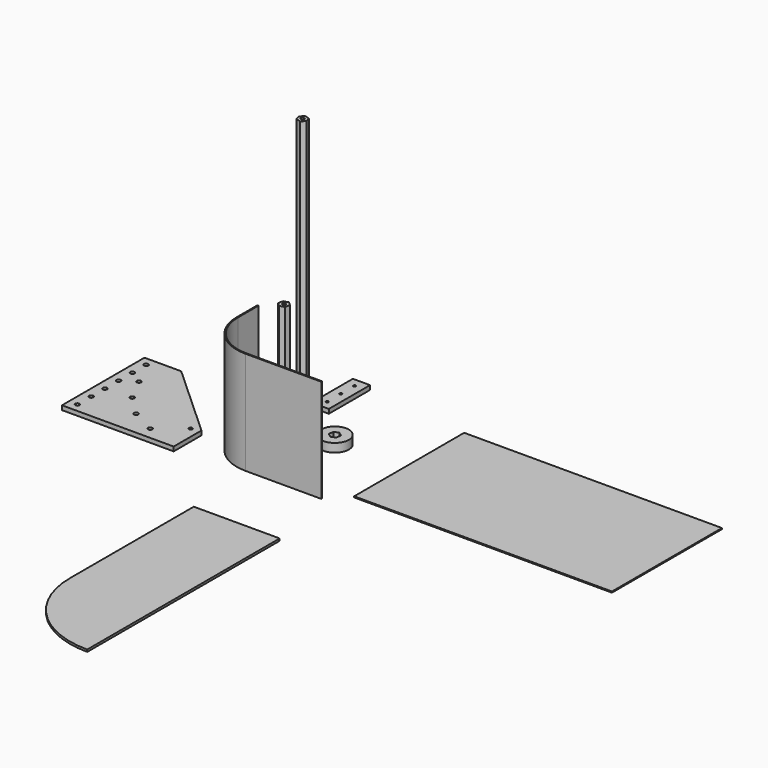
from build123d import *

# Parameters (mm, degrees)
F0_W      = 25.4
F0_H      = 76.2
F0_R      = 1.905
F1_DEPTH  = 6.35
F2_W      = 381
F2_H      = 203.2
F3_DEPTH  = 1.5875
F4_R      = 3.175
F4_R_2    = 2.54
F5_DEPTH  = 6.35
F7_DEPTH  = 3.175
F8_R      = 2.5527
F9_DEPTH  = 155.575
F11_DEPTH = 152.4
F12_R     = 2.5527
F13_DEPTH = 406.4
F14_R     = 20.6375
F15_DEPTH = 12.7


# Not quite as in the source:
# - a length typed as a fraction of an inch, garbled in the dataset ("3 / 203.2 mm" for 3/8 in), is restored


with BuildPart() as f1:
    # F0 (on Top) → F1 (new body)
    with BuildSketch(Plane.XY):
        with Locations((-43.9476225885, 36.8518919408)):
            Rectangle(F0_W, F0_H)
        with Locations((-43.9476225885, 11.4518919408)):
            Circle(F0_R, mode=Mode.SUBTRACT)
        with Locations((-43.9476225885, 36.8518919408)):
            Circle(F0_R, mode=Mode.SUBTRACT)
        with Locations((-43.9476225885, 62.2518919408)):
            Circle(F0_R, mode=Mode.SUBTRACT)
    extrude(amount=F1_DEPTH)


with BuildPart() as f3:
    # F2 (on Top) → F3 (new body)
    with BuildSketch(Plane.XY):
        with Locations((312.7722548485, -44.6919236064)):
            Rectangle(F2_W, F2_H)
    extrude(amount=F3_DEPTH)


with BuildPart() as f5:
    # F4 (on Top) → F5 (new body)
    with BuildSketch(Plane.XY):
        Polygon((-223.0699211359, -34.1322505951), (-277.4203166646, -34.1322505951), (-277.4203166646, -186.5322505951), (-112.3203166646, -186.5322505951), (-112.3203166646, -135.2008368701), align=None)
        with Locations((-264.7203166646, -173.8322505951)):
            Circle(F4_R, mode=Mode.SUBTRACT)
        with Locations((-197.4012885681, -149.550242086)):
            Circle(F4_R, mode=Mode.SUBTRACT)
        with Locations((-264.7203166646, -148.4322505951)):
            Circle(F4_R, mode=Mode.SUBTRACT)
        with Locations((-264.7203166646, -123.0322505951)):
            Circle(F4_R, mode=Mode.SUBTRACT)
        with Locations((-226.1381081555, -120.8134224986)):
            Circle(F4_R, mode=Mode.SUBTRACT)
        with Locations((-161.433759699, -168.4697153093)):
            Circle(F4_R, mode=Mode.SUBTRACT)
        with Locations((-125.0203166646, -139.3370777369)):
            Circle(F4_R_2, mode=Mode.SUBTRACT)
        with Locations((-264.7203166646, -97.6322505951)):
            Circle(F4_R, mode=Mode.SUBTRACT)
        with Locations((-245.0575813788, -84.8458936294)):
            Circle(F4_R, mode=Mode.SUBTRACT)
        with Locations((-264.7203166646, -72.2322505951)):
            Circle(F4_R, mode=Mode.SUBTRACT)
        with Locations((-264.7203166646, -46.8322505951)):
            Circle(F4_R, mode=Mode.SUBTRACT)
    extrude(amount=F5_DEPTH)


with BuildPart() as f7:
    # F6 (on Top) → F7 (new body)
    with BuildSketch(Plane.XY):
        with BuildLine():
            Line((122.8882094549, -284.6549875146), (-4.1117905451, -284.6549875146))
            Line((-4.1117905451, -284.6549875146), (-4.1117905451, -513.2549875146))
            ThreePointArc((-4.1117905451, -513.2549875146), (33.0856482442, -603.0575487253), (122.8882094549, -640.2549875146))
            Line((122.8882094549, -640.2549875146), (122.8882094549, -513.2549875146))
            Line((122.8882094549, -513.2549875146), (122.8882094549, -284.6549875146))
        make_face()
    extrude(amount=F7_DEPTH)


with BuildPart() as f9:
    # F8 (on Top) → F9 (new body)
    with BuildSketch(Plane.XY):
        Polygon((-57.9077300241, -59.8681378041), (-50.8764464785, -57.7886222274), (-49.1617180227, -50.6595942672), (-54.4782731125, -45.6100818839), (-61.5095566582, -47.6895974606), (-63.224285114, -54.8186254207), align=None)
        with Locations((-56.1930015683, -52.739109844)):
            Circle(F8_R, mode=Mode.SUBTRACT)
    extrude(amount=F9_DEPTH)


with BuildPart() as f11:
    # F10 (on Top) → F11 (new body)
    with BuildSketch(Plane.XY):
        with BuildLine():
            ThreePointArc((-17.1079281718, -171.1775491238), (-62.0092087771, -152.5788297291), (-80.6079281718, -107.6775491238))
            Line((-80.6079281718, -107.6775491238), (-80.6079281718, -69.5775491238))
            Line((-80.6079281718, -69.5775491238), (-82.1954281718, -69.5775491238))
            Line((-82.1954281718, -69.5775491238), (-82.1954281718, -107.6775491238))
            ThreePointArc((-82.1954281718, -107.6775491238), (-63.1317407922, -153.7013617442), (-17.1079281718, -172.7650491238))
            Line((-17.1079281718, -172.7650491238), (94.8303937912, -172.7650491238))
            Line((94.8303937912, -172.7650491238), (94.8303937912, -171.1775491238))
            Line((94.8303937912, -171.1775491238), (-17.1079281718, -171.1775491238))
        make_face()
    extrude(amount=F11_DEPTH)


with BuildPart() as f13:
    # F12 (on Top) → F13 (new body)
    with BuildSketch(Plane.XY):
        Polygon((-25.9567694114, -60.8674003933), (-20.7720161226, -55.6826471044), (-22.6697675386, -48.6001423994), (-29.7522722436, -46.7023909833), (-34.9370255325, -51.8871442722), (-33.0392741164, -58.9696489772), align=None)
        with Locations((-27.8545208275, -53.7848956883)):
            Circle(F12_R, mode=Mode.SUBTRACT)
    extrude(amount=F13_DEPTH)


with BuildPart() as f15:
    # F14 (on Top) → F15 (new body)
    with BuildSketch(Plane.XY):
        with Locations((22.1018530428, -56.7118227482)):
            Circle(F14_R)
        Polygon((28.8261292295, -53.7882216984), (27.9959039159, -61.073416223), (21.2716277292, -63.9970172728), (15.3775768562, -59.635423798), (16.2078021698, -52.3502292734), (22.9320783565, -49.4266282235), align=None, mode=Mode.SUBTRACT)
    extrude(amount=F15_DEPTH)


solid = Compound([f1.part, f3.part, f5.part, f7.part, f9.part, f11.part, f13.part, f15.part])
